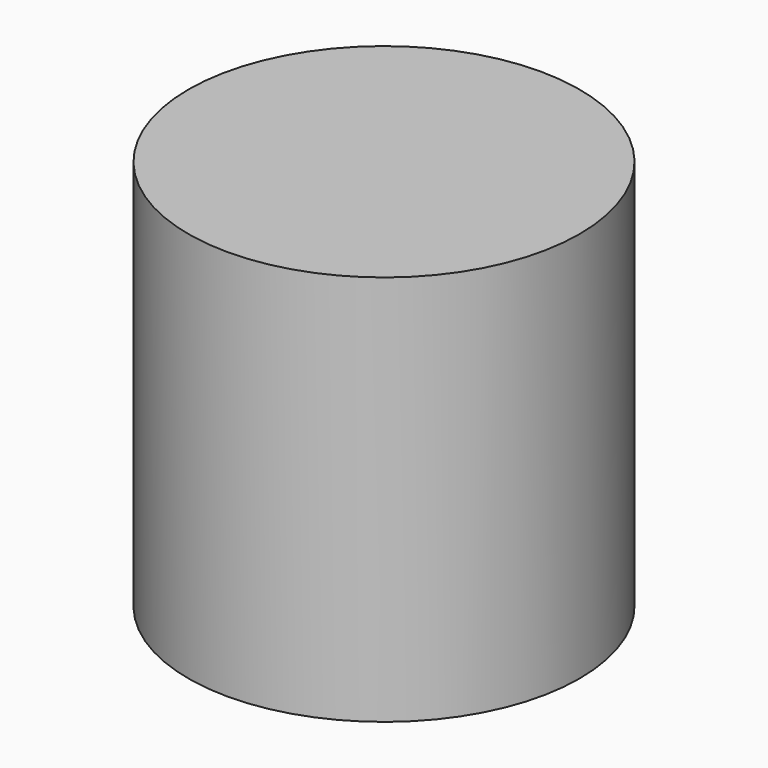
from build123d import *

# Parameters (mm, degrees)
F0_R     = 12.7
F0_R_2   = 9.525
F2_DEPTH = 25.4


# Not quite as in the source:
# - a variable given as a bare number and used for a length is read in inches; the dataset says mm whatever the document's units were


with BuildPart() as f2:
    # F0 (on Top) → F2 (new body)
    with BuildSketch(Plane.XY):
        Circle(F0_R)
        Circle(F0_R_2, mode=Mode.SUBTRACT)
        Circle(F0_R_2)
    extrude(amount=F2_DEPTH)


solid = f2.part
